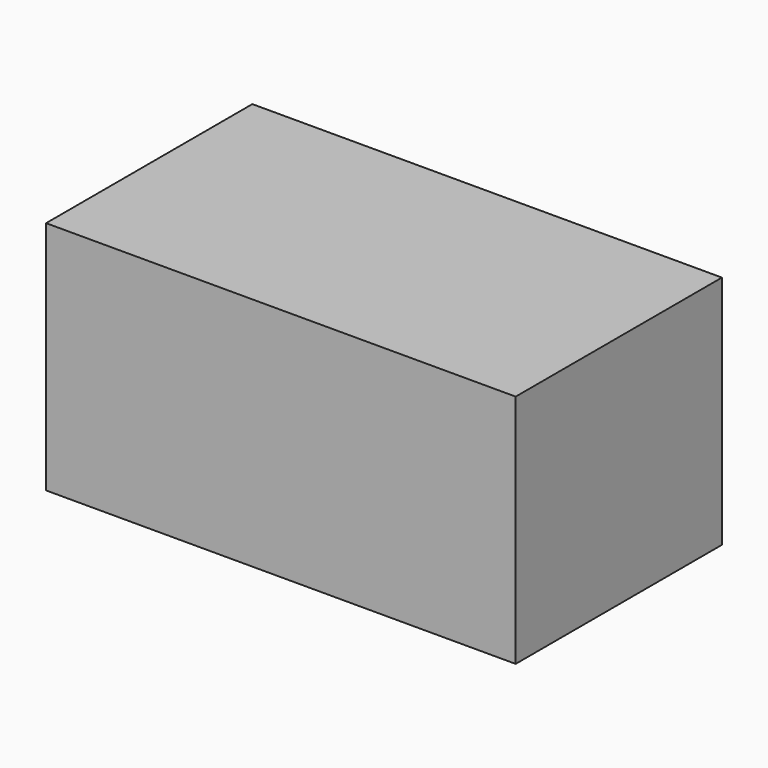
from build123d import *

# Parameters (mm, degrees)
F0_W         = 49.8913060874
F0_H         = 27.3913051933
F0_TEXT_SIZE = 4.981883103
F1_DEPTH     = 25


# Not quite as in the source:
# - Text() gives the source's letters only with a copy of the font that has no kerning and outlines rounded to 1/6400 em; it was checked with that copy


with BuildPart() as f1:
    # F0 (on Top) → F1 (new body)
    with BuildSketch(Plane.XY):
        with Locations((3.2608686015, -0.326086767)):
            Rectangle(F0_W, F0_H)
        Polygon((3.641727586, -6.5217399679), (3.2135970068, -6.5217399679), (2.7706764622, -5.3906968196), (1.3453908432, -5.3906968196), (0.9079192332, -6.5217399679), (0.4891296849, -6.5217399679), (1.894954823, -2.9503525184), (2.242908221, -2.9503525184), align=None, mode=Mode.SUBTRACT)
        with BuildLine():
            add(Edge.make_bspline(
                [(5.6228045387, -5.3541111156), (5.7893862549, -5.5292554434), (5.7893862549, -5.7946964025)],
                knots=[0, 0, 0, 1, 1, 1], degree=2))
            add(Edge.make_bspline(
                [(5.7893862549, -5.7946964025), (5.7893862549, -6.1667807968), (5.5122690073, -6.3687805882)],
                knots=[0, 0, 0, 1, 1, 1], degree=2))
            add(Edge.make_bspline(
                [(5.5122690073, -6.3687805882), (5.2351517597, -6.5707803797), (4.7338497725, -6.5707803797)],
                knots=[0, 0, 0, 1, 1, 1], degree=2))
            add(Edge.make_bspline(
                [(4.7338497725, -6.5707803797), (4.2037462736, -6.5707803797), (3.9071685451, -6.4026418249)],
                knots=[0, 0, 0, 1, 1, 1], degree=2))
            Line((3.9071685451, -6.4026418249), (3.9071685451, -6.028222173))
            add(Edge.make_bspline(
                [(3.9071685451, -6.028222173), (4.0994380961, -6.1255245773), (4.3193415299, -6.1811815526)],
                knots=[0, 0, 0, 1, 1, 1], degree=2))
            add(Edge.make_bspline(
                [(4.3193415299, -6.1811815526), (4.5392449638, -6.2368385279), (4.7439692225, -6.2368385279)],
                knots=[0, 0, 0, 1, 1, 1], degree=2))
            add(Edge.make_bspline(
                [(4.7439692225, -6.2368385279), (5.0600074319, -6.2368385279), (5.2300920347, -6.136033237)],
                knots=[0, 0, 0, 1, 1, 1], degree=2))
            add(Edge.make_bspline(
                [(5.2300920347, -6.136033237), (5.4001766375, -6.0352279461), (5.4001766375, -5.8281684296)],
                knots=[0, 0, 0, 1, 1, 1], degree=2))
            add(Edge.make_bspline(
                [(5.4001766375, -5.8281684296), (5.4001766375, -5.6724845826), (5.2655101099, -5.5619490513)],
                knots=[0, 0, 0, 1, 1, 1], degree=2))
            add(Edge.make_bspline(
                [(5.2655101099, -5.5619490513), (5.1308435823, -5.4514135199), (4.7385202879, -5.3004001884)],
                knots=[0, 0, 0, 1, 1, 1], degree=2))
            add(Edge.make_bspline(
                [(4.7385202879, -5.3004001884), (4.3664358936, -5.1618415646), (4.2095844178, -5.0583118064)],
                knots=[0, 0, 0, 1, 1, 1], degree=2))
            add(Edge.make_bspline(
                [(4.2095844178, -5.0583118064), (4.052732942, -4.9547820481), (3.9760586474, -4.823618407)],
                knots=[0, 0, 0, 1, 1, 1], degree=2))
            add(Edge.make_bspline(
                [(3.9760586474, -4.823618407), (3.8993843527, -4.692454766), (3.8993843527, -4.510304665)],
                knots=[0, 0, 0, 1, 1, 1], degree=2))
            add(Edge.make_bspline(
                [(3.8993843527, -4.510304665), (3.8993843527, -4.1841470056), (4.1648253118, -3.9953803412)],
                knots=[0, 0, 0, 1, 1, 1], degree=2))
            add(Edge.make_bspline(
                [(4.1648253118, -3.9953803412), (4.4302662709, -3.8066136767), (4.8918688772, -3.8066136767)],
                knots=[0, 0, 0, 1, 1, 1], degree=2))
            add(Edge.make_bspline(
                [(4.8918688772, -3.8066136767), (5.322334714, -3.8066136767), (5.7341184893, -3.9817580046)],
                knots=[0, 0, 0, 1, 1, 1], degree=2))
            Line((5.7341184893, -3.9817580046), (5.5901109308, -4.3102509217))
            add(Edge.make_bspline(
                [(5.5901109308, -4.3102509217), (5.1892250249, -4.1452260439), (4.8630673655, -4.1452260439)],
                knots=[0, 0, 0, 1, 1, 1], degree=2))
            add(Edge.make_bspline(
                [(4.8630673655, -4.1452260439), (4.5758306678, -4.1452260439), (4.4298770613, -4.2351334655)],
                knots=[0, 0, 0, 1, 1, 1], degree=2))
            add(Edge.make_bspline(
                [(4.4298770613, -4.2351334655), (4.2839234548, -4.3250408871), (4.2839234548, -4.4830599918)],
                knots=[0, 0, 0, 1, 1, 1], degree=2))
            add(Edge.make_bspline(
                [(4.2839234548, -4.4830599918), (4.2839234548, -4.5904818462), (4.3388020108, -4.6655993024)],
                knots=[0, 0, 0, 1, 1, 1], degree=2))
            add(Edge.make_bspline(
                [(4.3388020108, -4.6655993024), (4.3936805669, -4.7407167585), (4.5151139675, -4.8088284416)],
                knots=[0, 0, 0, 1, 1, 1], degree=2))
            add(Edge.make_bspline(
                [(4.5151139675, -4.8088284416), (4.6365473681, -4.8769401246), (4.9821655084, -5.0061577176)],
                knots=[0, 0, 0, 1, 1, 1], degree=2))
            add(Edge.make_bspline(
                [(4.9821655084, -5.0061577176), (5.4562228224, -5.1789667878), (5.6228045387, -5.3541111156)],
                knots=[0, 0, 0, 1, 1, 1], degree=2))
        make_face(mode=Mode.SUBTRACT)
        with BuildLine():
            Line((8.6749863585, -6.5217399679), (8.2709867756, -6.5217399679))
            Line((8.2709867756, -6.5217399679), (8.2709867756, -4.7967629434))
            add(Edge.make_bspline(
                [(8.2709867756, -4.7967629434), (8.2709867756, -4.4713837033), (8.1226979114, -4.3106401313)],
                knots=[0, 0, 0, 1, 1, 1], degree=2))
            add(Edge.make_bspline(
                [(8.1226979114, -4.3106401313), (7.9744090472, -4.1498965593), (7.6575924186, -4.1498965593)],
                knots=[0, 0, 0, 1, 1, 1], degree=2))
            add(Edge.make_bspline(
                [(7.6575924186, -4.1498965593), (7.2372460318, -4.1498965593), (7.0438088519, -4.3787518143)],
                knots=[0, 0, 0, 1, 1, 1], degree=2))
            add(Edge.make_bspline(
                [(7.0438088519, -4.3787518143), (6.850371672, -4.6076070694), (6.850371672, -5.1275911183)],
                knots=[0, 0, 0, 1, 1, 1], degree=2))
            Line((6.850371672, -5.1275911183), (6.850371672, -6.5217399679))
            Line((6.850371672, -6.5217399679), (6.4463720892, -6.5217399679))
            Line((6.4463720892, -6.5217399679), (6.4463720892, -2.7362872288))
            Line((6.4463720892, -2.7362872288), (6.850371672, -2.7362872288))
            Line((6.850371672, -2.7362872288), (6.850371672, -3.8821203425))
            add(Edge.make_bspline(
                [(6.850371672, -3.8821203425), (6.850371672, -4.089179859), (6.8309111912, -4.2254032251)],
                knots=[0, 0, 0, 1, 1, 1], degree=2))
            Line((6.8309111912, -4.2254032251), (6.8550421875, -4.2254032251))
            add(Edge.make_bspline(
                [(6.8550421875, -4.2254032251), (6.9741403304, -4.0331336741), (7.1944329738, -3.9225981427)],
                knots=[0, 0, 0, 1, 1, 1], degree=2))
            add(Edge.make_bspline(
                [(7.1944329738, -3.9225981427), (7.4147256173, -3.8120626114), (7.6965133803, -3.8120626114)],
                knots=[0, 0, 0, 1, 1, 1], degree=2))
            add(Edge.make_bspline(
                [(7.6965133803, -3.8120626114), (8.1853606598, -3.8120626114), (8.4301735092, -4.044420753)],
                knots=[0, 0, 0, 1, 1, 1], degree=2))
            add(Edge.make_bspline(
                [(8.4301735092, -4.044420753), (8.6749863585, -4.2767788946), (8.6749863585, -4.7827513972)],
                knots=[0, 0, 0, 1, 1, 1], degree=2))
            Line((8.6749863585, -4.7827513972), (8.6749863585, -6.5217399679))
        make_face(mode=Mode.SUBTRACT)
        with BuildLine():
            Line((9.475201332, -3.8556540885), (9.8838714302, -3.8556540885))
            Line((9.8838714302, -3.8556540885), (9.8838714302, -5.5853016283))
            add(Edge.make_bspline(
                [(9.8838714302, -5.5853016283), (9.8838714302, -5.9114592877), (10.0321602945, -6.0718136501)],
                knots=[0, 0, 0, 1, 1, 1], degree=2))
            add(Edge.make_bspline(
                [(10.0321602945, -6.0718136501), (10.1804491587, -6.2321680125), (10.4964873681, -6.2321680125)],
                knots=[0, 0, 0, 1, 1, 1], degree=2))
            add(Edge.make_bspline(
                [(10.4964873681, -6.2321680125), (10.9152769164, -6.2321680125), (11.1083248867, -6.0037019671)],
                knots=[0, 0, 0, 1, 1, 1], degree=2))
            add(Edge.make_bspline(
                [(11.1083248867, -6.0037019671), (11.3013728569, -5.7752359216), (11.3013728569, -5.2568087112)],
                knots=[0, 0, 0, 1, 1, 1], degree=2))
            Line((11.3013728569, -5.2568087112), (11.3013728569, -3.8556540885))
            Line((11.3013728569, -3.8556540885), (11.7053724398, -3.8556540885))
            Line((11.7053724398, -3.8556540885), (11.7053724398, -6.5217399679))
            Line((11.7053724398, -6.5217399679), (11.3722090073, -6.5217399679))
            Line((11.3722090073, -6.5217399679), (11.3138275647, -6.1644455391))
            Line((11.3138275647, -6.1644455391), (11.2920318261, -6.1644455391))
            add(Edge.make_bspline(
                [(11.2920318261, -6.1644455391), (11.1682631677, -6.3613856055), (10.9479705243, -6.4660829926)],
                knots=[0, 0, 0, 1, 1, 1], degree=2))
            add(Edge.make_bspline(
                [(10.9479705243, -6.4660829926), (10.7276778808, -6.5707803797), (10.4451116986, -6.5707803797)],
                knots=[0, 0, 0, 1, 1, 1], degree=2))
            add(Edge.make_bspline(
                [(10.4451116986, -6.5707803797), (9.9585996768, -6.5707803797), (9.7169005044, -6.3395898669)],
                knots=[0, 0, 0, 1, 1, 1], degree=2))
            add(Edge.make_bspline(
                [(9.7169005044, -6.3395898669), (9.475201332, -6.1083993542), (9.475201332, -5.6000915938)],
                knots=[0, 0, 0, 1, 1, 1], degree=2))
            Line((9.475201332, -5.6000915938), (9.475201332, -3.8556540885))
        make_face(mode=Mode.SUBTRACT)
        with BuildLine():
            Line((1.4917336593, -5.0186124254), (2.6422372885, -5.0186124254))
            Line((2.6422372885, -5.0186124254), (2.2281182555, -3.9163707888))
            add(Edge.make_bspline(
                [(2.2281182555, -3.9163707888), (2.1479410743, -3.7069760147), (2.0630933777, -3.4033925131)],
                knots=[0, 0, 0, 1, 1, 1], degree=2))
            add(Edge.make_bspline(
                [(2.0630933777, -3.4033925131), (2.0093824505, -3.6369182835), (1.9097447885, -3.9163707888)],
                knots=[0, 0, 0, 1, 1, 1], degree=2))
            Line((1.9097447885, -3.9163707888), (1.4917336593, -5.0186124254))
        make_face()
        with Locations((0.4891296849, -6.5217399679)):
            Text('Ashu', F0_TEXT_SIZE, font='Open Sans', text_align=(TextAlign.LEFT, TextAlign.BOTTOM))
    extrude(amount=F1_DEPTH)


solid = f1.part
